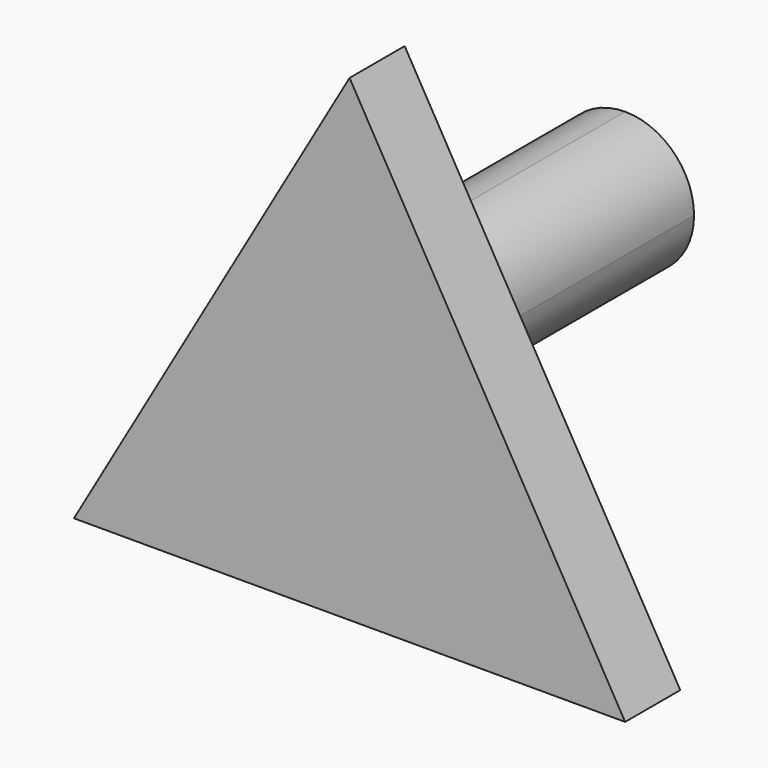
from build123d import *

# Parameters (mm, degrees)
F1_DEPTH = 5
F3_DEPTH = 25


with BuildPart() as f1:
    # F0 (on Front) → F1 (new body)
    with BuildSketch(Plane.XZ):
        Polygon((-20, 0), (0, 0), (20, 0), (0, 34.6410161514), align=None)
    extrude(amount=F1_DEPTH)

    # F2 (on face) → F3 (join)
    with BuildSketch(Plane.XZ.offset(5)):
        with BuildLine():
            Line((0, 22.3205080757), (0, 12.3205080757))
            ThreePointArc((0, 12.3205080757), (3.5355339059, 13.7849741698), (5, 17.3205080757))
            ThreePointArc((5, 17.3205080757), (3.5355339059, 20.8560419816), (0, 22.3205080757))
        make_face()
        with BuildLine():
            ThreePointArc((0, 22.3205080757), (-5, 17.3205080757), (0, 12.3205080757))
            Line((0, 12.3205080757), (0, 22.3205080757))
        make_face()
    extrude(amount=-F3_DEPTH)


solid = f1.part
